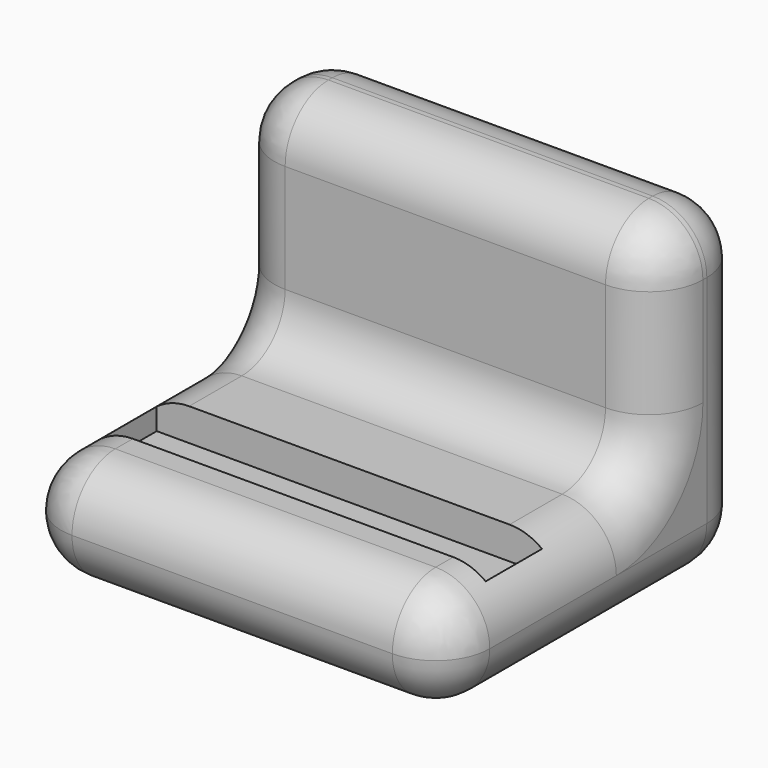
from build123d import *

# Parameters (mm, degrees)
F0_W         = 100.5891636014
F0_H         = 89.0790522099
F1_DEPTH     = 25.4
F2_W         = 100.5891636014
F2_H         = 26.5494063497
F3_DEPTH     = 50.8
F4_W         = 90.4291636014
F4_H         = 16.5267549455
F5_DEPTH     = 7.62
F6_F1_R      = 12.7
F6_F2_R      = 12.6999
F6_T3_DEPTH  = 49.8296458602
F6_T5_DEPTH  = 38.1
F6_T8_ANGLE  = 90
F6_T10_ANGLE = 90
F6_T12_ANGLE = 90
F6_T14_ANGLE = 90
F6_T16_ANGLE = 90
F6_T18_ANGLE = 90


# Not quite as in the source:
# - a fillet or chamfer that OpenCascade refuses, or shapes differently, is made with other operations: its cross-section is extruded or revolved along the edge and cut away or added
# - a fillet or chamfer is up to 0.001 mm smaller than in the source, because OpenCascade refuses the exact size


with BuildPart() as f1:
    # F0 (on Top) → F1 (new body)
    with BuildSketch(Plane.XY):
        with Locations((1.1365450919, 10.1573467255)):
            Rectangle(F0_W, F0_H)
    extrude(amount=F1_DEPTH)

    # F2 (on face) → F3 (join)
    with BuildSketch(Plane.XY.offset(25.4)):
        with Locations((1.1365450919, 41.4221696556)):
            Rectangle(F2_W, F2_H)
    extrude(amount=F3_DEPTH)

    # F4 (on face) → F5 (cut)
    with BuildSketch(Plane.XY.offset(25.4)):
        with Locations((1.1365450919, -8.2633774728)):
            Rectangle(F4_W, F4_H)
    extrude(amount=-F5_DEPTH, mode=Mode.SUBTRACT)

    # F6: fillet of radius 12.7 on 18 edges, made by hand

    # F6_f1
    f6_f1_edges = [f1.edges().sort_by_distance(p)[0] for p in [
        (1.1365450919, 28.1474664807, 25.4),
    ]]
    fillet(f6_f1_edges, radius=F6_F1_R)

    # F6_f2 (radius 12.7 in the source; OpenCascade refuses exactly that, so slightly less here)
    f6_f2_edges = [f1.edges().sort_by_distance(p)[0] for p in [
        (1.1365450919, -34.3821793795, 25.4),
        (51.4311268926, -34.3821793795, 12.7),
        (1.1365450919, -34.3821793795, 0),
        (-49.1580367088, -34.3821793795, 12.7),
        (1.1365450919, 28.1474664807, 76.2),
        (51.4311268926, 10.1573467255, 0),
        (51.4311268926, 54.6968728304, 38.1),
        (51.4311268926, 41.4221696556, 76.2),
        (1.1365450919, 54.6968728304, 76.2),
        (-49.1580367088, 41.4221696556, 76.2),
        (-49.1580367088, 10.1573467255, 0),
        (-49.1580367088, 54.6968728304, 38.1),
        (1.1365450919, 54.6968728304, 0),
    ]]
    fillet(f6_f2_edges, radius=F6_F2_R)

    # F6_s4 → F6_t3 (cut)
    with BuildSketch(Plane.XZ.offset(-15.4474664807)):
        with BuildLine():
            ThreePointArc((-49.1580367088, 12.7), (-45.4382928299, 21.6802561211), (-36.4580367088, 25.4))
            Line((-36.4580367088, 25.4), (-36.4580367088, 25.654))
            Line((-36.4580367088, 25.654), (-49.4120367088, 25.654))
            Line((-49.4120367088, 25.654), (-49.4120367088, 12.7))
            Line((-49.4120367088, 12.7), (-49.1580367088, 12.7))
        make_face()
        with BuildLine():
            ThreePointArc((38.7311268926, 25.4), (47.7113830136, 21.6802561211), (51.4311268926, 12.7))
            Line((51.4311268926, 12.7), (51.6851268926, 12.7))
            Line((51.6851268926, 12.7), (51.6851268926, 25.654))
            Line((51.6851268926, 25.654), (38.7311268926, 25.654))
            Line((38.7311268926, 25.654), (38.7311268926, 25.4))
        make_face()
    extrude(amount=F6_T3_DEPTH, mode=Mode.SUBTRACT)

    # F6_s6 → F6_t5 (cut)
    with BuildSketch(Plane.XY.offset(38.1)):
        with BuildLine():
            ThreePointArc((-49.1580367088, 40.8474664807), (-45.4382928299, 31.8672103597), (-36.4580367088, 28.1474664807))
            Line((-36.4580367088, 28.1474664807), (-36.4580367088, 27.8934664807))
            Line((-36.4580367088, 27.8934664807), (-49.4120367088, 27.8934664807))
            Line((-49.4120367088, 27.8934664807), (-49.4120367088, 40.8474664807))
            Line((-49.4120367088, 40.8474664807), (-49.1580367088, 40.8474664807))
        make_face()
        with BuildLine():
            ThreePointArc((38.7311268926, 28.1474664807), (47.7113830136, 31.8672103597), (51.4311268926, 40.8474664807))
            Line((51.4311268926, 40.8474664807), (51.6851268926, 40.8474664807))
            Line((51.6851268926, 40.8474664807), (51.6851268926, 27.8934664807))
            Line((51.6851268926, 27.8934664807), (38.7311268926, 27.8934664807))
            Line((38.7311268926, 27.8934664807), (38.7311268926, 28.1474664807))
        make_face()
    extrude(amount=F6_T5_DEPTH, mode=Mode.SUBTRACT)

    # F6_s7 → F6_t8 (revolve, cut)
    with BuildSketch(Plane.XY.offset(12.7)):
        with BuildLine():
            ThreePointArc((38.7312268926, -34.3821793795), (47.711412303, -30.6624647899), (51.4311268926, -21.6822793795))
            Line((51.4311268926, -21.6822793795), (51.4311268926, -34.3821793795))
            Line((51.4311268926, -34.3821793795), (38.7312268926, -34.3821793795))
        make_face()
    revolve(axis=Axis((38.7311268926, -34.3821793795, 12.7), (0, -1, 0)), revolution_arc=F6_T8_ANGLE, mode=Mode.SUBTRACT)

    # F6_s9 → F6_t10 (revolve, cut)
    with BuildSketch(Plane.YZ.offset(38.7311268926)):
        with BuildLine():
            ThreePointArc((40.8473664807, 76.2), (31.8671810703, 72.4802854104), (28.1474664807, 63.5001))
            Line((28.1474664807, 63.5001), (28.1474664807, 76.2))
            Line((28.1474664807, 76.2), (40.8473664807, 76.2))
        make_face()
    revolve(axis=Axis((38.7311268926, 40.8474664807, 76.2), (0, 0, 1)), revolution_arc=F6_T10_ANGLE, mode=Mode.SUBTRACT)

    # F6_s11 → F6_t12 (revolve, cut)
    with BuildSketch(Plane.XZ.offset(-40.8474664807)):
        with BuildLine():
            ThreePointArc((-36.4581367088, 76.2), (-45.4383221192, 72.4802854104), (-49.1580367088, 63.5001))
            Line((-49.1580367088, 63.5001), (-49.1580367088, 76.2))
            Line((-49.1580367088, 76.2), (-36.4581367088, 76.2))
        make_face()
    revolve(axis=Axis((-36.4580367088, 40.8474664807, 76.2), (0, 0, 1)), revolution_arc=F6_T12_ANGLE, mode=Mode.SUBTRACT)

    # F6_s13 → F6_t14 (revolve, cut)
    with BuildSketch(Plane.YZ.offset(-36.4580367088)):
        with BuildLine():
            ThreePointArc((-34.3821793795, 12.7001), (-30.6624647899, 21.6802854104), (-21.6822793795, 25.4))
            Line((-21.6822793795, 25.4), (-34.3821793795, 25.4))
            Line((-34.3821793795, 25.4), (-34.3821793795, 12.7001))
        make_face()
    revolve(axis=Axis((-36.4580367088, -34.3821793795, 12.7), (0, -1, 0)), revolution_arc=F6_T14_ANGLE, mode=Mode.SUBTRACT)

    # F6_s15 → F6_t16 (revolve, cut)
    with BuildSketch(Plane.XY.offset(38.1)):
        with BuildLine():
            ThreePointArc((38.7311268926, 28.1474664807), (47.7113830136, 31.8672103597), (51.4311268926, 40.8474664807))
            Line((51.4311268926, 40.8474664807), (51.6851268926, 40.8474664807))
            Line((51.6851268926, 40.8474664807), (51.6851268926, 27.8934664807))
            Line((51.6851268926, 27.8934664807), (38.7311268926, 27.8934664807))
            Line((38.7311268926, 27.8934664807), (38.7311268926, 28.1474664807))
        make_face()
    revolve(axis=Axis((51.4311268926, 15.4474664807, 38.1), (-1, 0, 0)), revolution_arc=F6_T16_ANGLE, mode=Mode.SUBTRACT)

    # F6_s17 → F6_t18 (revolve, cut)
    with BuildSketch(Plane.XY.offset(38.1)):
        with BuildLine():
            ThreePointArc((-49.1580367088, 40.8474664807), (-45.4382928299, 31.8672103597), (-36.4580367088, 28.1474664807))
            Line((-36.4580367088, 28.1474664807), (-36.4580367088, 27.8934664807))
            Line((-36.4580367088, 27.8934664807), (-49.4120367088, 27.8934664807))
            Line((-49.4120367088, 27.8934664807), (-49.4120367088, 40.8474664807))
            Line((-49.4120367088, 40.8474664807), (-49.1580367088, 40.8474664807))
        make_face()
    revolve(axis=Axis((-49.1580367088, 15.4474664807, 38.1), (-1, 0, 0)), revolution_arc=F6_T18_ANGLE, mode=Mode.SUBTRACT)


solid = f1.part
